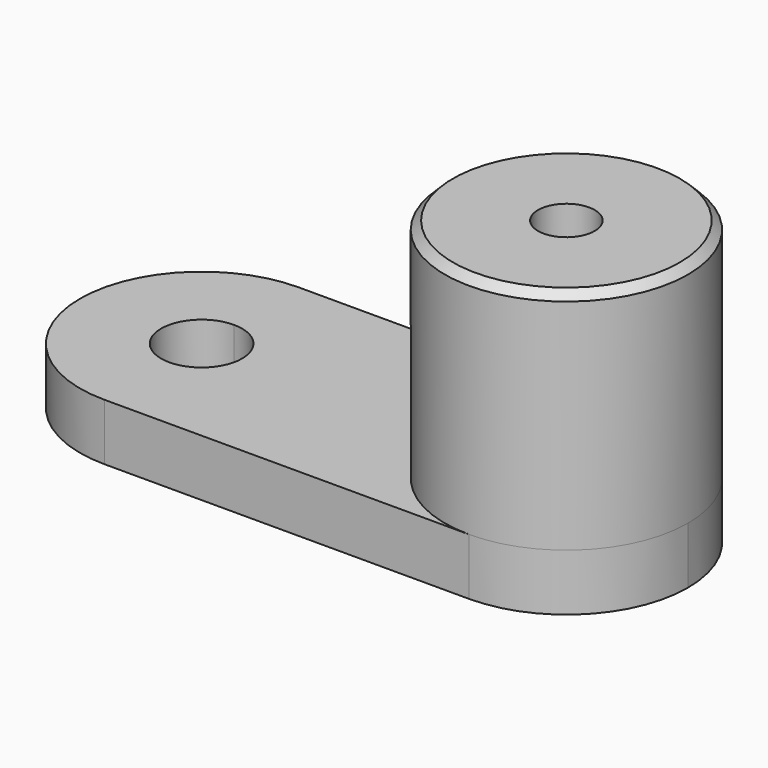
from build123d import *

# Parameters (mm, degrees)
F1_DEPTH = 7
F2_R     = 15
F2_R_2   = 8.25
F3_DEPTH = 22
F4_R     = 15
F4_R_2   = 3.5
F5_DEPTH = 6
F6_SIZE2 = 1
F6_SIZE  = 1


with BuildPart() as f1:
    # F0 (on Top) → F1 (new body)
    with BuildSketch(Plane.XY):
        with BuildLine():
            ThreePointArc((-22.5, -15), (-11.893398, -10.606602), (-7.5, 0))
            ThreePointArc((-7.5, 0), (-11.893398, 10.606602), (-22.5, 15))
            Line((-22.5, 15), (-22.5, 5))
            ThreePointArc((-22.5, 5), (-18.964466, 3.535534), (-17.5, 0))
            ThreePointArc((-17.5, 0), (-18.964466, -3.535534), (-22.5, -5))
            Line((-22.5, -5), (-22.5, -15))
        make_face()
        with BuildLine():
            ThreePointArc((-22.5, 15), (-11.893398, 10.606602), (-7.5, 0))
            ThreePointArc((-7.5, 0), (-11.893398, -10.606602), (-22.5, -15))
            Line((-22.5, -15), (22.5, -15))
            ThreePointArc((22.5, -15), (7.5, 0), (22.5, 15))
            Line((22.5, 15), (-22.5, 15))
        make_face()
        with BuildLine():
            Line((-22.5, 5), (-22.5, 15))
            ThreePointArc((-22.5, 15), (-37.5, 0), (-22.5, -15))
            Line((-22.5, -15), (-22.5, -5))
            ThreePointArc((-22.5, -5), (-27.5, 0), (-22.5, 5))
        make_face()
        with BuildLine():
            Line((22.5, 8.25), (22.5, 15))
            ThreePointArc((22.5, 15), (7.5, 0), (22.5, -15))
            Line((22.5, -15), (22.5, -8.25))
            ThreePointArc((22.5, -8.25), (14.25, 0), (22.5, 8.25))
        make_face()
        with BuildLine():
            ThreePointArc((37.5, 0), (33.106602, 10.606602), (22.5, 15))
            Line((22.5, 15), (22.5, 8.25))
            ThreePointArc((22.5, 8.25), (28.333631, 5.833631), (30.75, 0))
            ThreePointArc((30.75, 0), (28.333631, -5.833631), (22.5, -8.25))
            Line((22.5, -8.25), (22.5, -15))
            ThreePointArc((22.5, -15), (33.106602, -10.606602), (37.5, 0))
        make_face()
    extrude(amount=F1_DEPTH)

    # F2 (on face) → F3 (join)
    with BuildSketch(Plane.XY.offset(7)):
        with Locations((22.5, 0)):
            Circle(F2_R)
        with Locations((22.5, 0)):
            Circle(F2_R_2, mode=Mode.SUBTRACT)
    extrude(amount=F3_DEPTH)

    # F4 (on face) → F5 (join)
    with BuildSketch(Plane.XY.offset(29)):
        with Locations((22.5, 0)):
            Circle(F4_R)
        with Locations((22.5, 0)):
            Circle(F4_R_2, mode=Mode.SUBTRACT)
    extrude(amount=F5_DEPTH)

    # F6
    f6_edges = [f1.edges().sort_by_distance(p)[0] for p in [
        (7.5, 0, 35),
    ]]
    chamfer(f6_edges, length=F6_SIZE, length2=F6_SIZE2)


solid = f1.part
